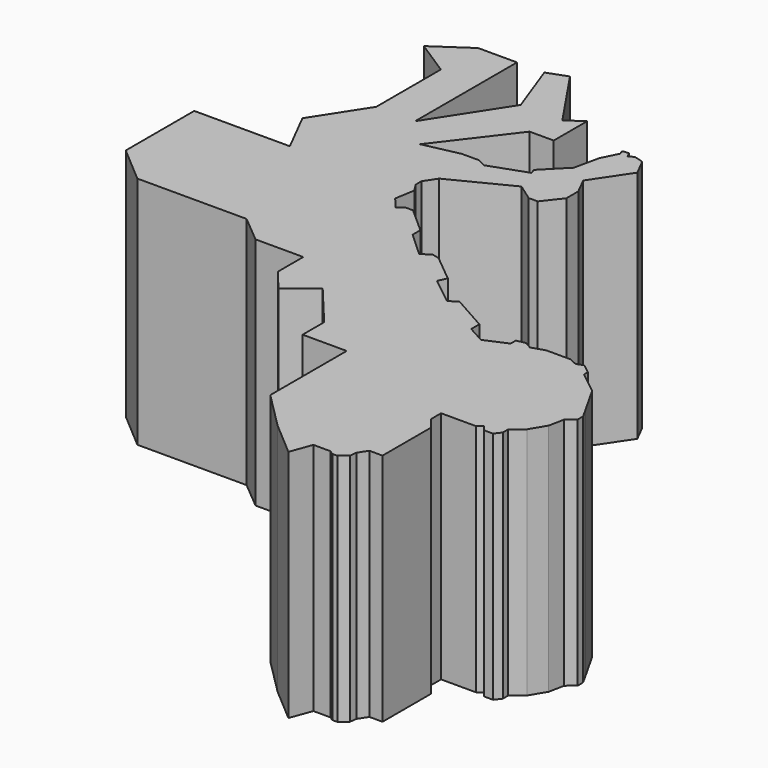
from build123d import *

# Parameters (mm, degrees)
F1_DEPTH    = 18.4
F2_T        = 1
F2_T3_DEPTH = 20.4


# Not quite as in the source:
# - a shell that OpenCascade refuses in one call is made with other operations: the cavity is built on its own and cut out


with BuildPart() as f1:
    # F0 (on Top) → F1 (new body)
    with BuildSketch(Plane.XY):
        Polygon((34.9038466811, 2.3076923098), (37.5961586833, 0), (38.2154919207, 1.6792200898), (39.5493015629, 1.6792200898), (39.8643054068, 1.4717115684), (40.2604434894, 1.4717115684), (40.8580452204, 1.969713252), (40.9277250636, 2.5216304831), (41.3846634328, 3.2152759377), (42.4140951151, 3.2152759377), (42.4140951151, 3.9669456892), (42.4140951151, 5.5783051066), (42.4140951151, 7.9888809662), (41.7042225599, 8.8407276198), (41.7042225599, 9.8502271683), (44.4576912096, 9.8502271683), (44.8243346239, 10.1557634948), (45.1803691685, 9.7285222481), (45.8762775312, 9.7285222481), (46.256152948, 10.2124772966), (46.256152948, 10.7373551534), (47.1577197313, 11.48866117), (47.8789657354, 12.6923089847), (48.1241039427, 13.9088267574), (48.7609393895, 14.4395232201), (48.7609393895, 14.9668920785), (48.3345761895, 15.7310124487), (47.0663927722, 17.9758262752), (45.3253550111, 19.3424355239), (45.3253550111, 19.7353474796), (44.5925742388, 20.310536027), (44.0478101373, 20.1109051704), (43.4293858707, 20.3982274979), (41.5340252221, 20.3982274979), (40.4943935573, 20.0712326914), (39.9509593844, 20.3926954418), (39.258543402, 20.2461257577), (39.258543402, 19.7353474796), (37.5306159258, 18.9858879894), (36.1601188779, 19.7353474796), (36.1601188779, 20.5363873392), (33.3506949246, 22.1185106784), (32.6812267303, 21.7167064548), (30.5281542242, 23.4213601798), (30.8408737183, 24.0895077586), (28.7077520043, 25.8446503431), (28.1511750072, 25.9745512158), (27.4442564696, 25.5241394043), (25.5313739181, 27.267659083), (25.5313739181, 28.0364025384), (23.5221236944, 29.8172839707), (22.9337685687, 29.8172839707), (22.4811825901, 29.4311344624), (21.6883961111, 30.3603187203), (21.9499040395, 31.9214127958), (21.5246956795, 32.5762294233), (21.5246956795, 33.1562906504), (22.1474349188, 34.1016265465), (26.7516728491, 36.4373363554), (28.0509851873, 35.5146564543), (28.7558529526, 35.5146564543), (29.8695010146, 36.9334258139), (29.8695010146, 38.1099569989), (29.2044375092, 39.4209548831), (31.1400774979, 42.3122339083), (30.4684508592, 43.6361692846), (29.7395295394, 43.846223038), (29.3254637787, 43.6361692846), (29.1439853609, 43.9939062825), (28.7558529526, 43.9939062825), (28.6115187719, 43.9206861825), (28.7558529526, 43.6361692846), (28.1240884215, 42.362369597), (27.6678408464, 40.2808707131), (27.4981055409, 40.1947647333), (25.9593750461, 38.6289927336), (26.0996799916, 38.2336303592), (23.197773844, 37.2038111091), (22.5049275905, 37.5358015299), (21.194729954, 37.5358015299), (18.3843486011, 36.9334258139), (22.5816704333, 42.4372814596), (24.4770020993, 42.4372814596), (24.4770020993, 45.7188370083), (23.2146158814, 44.8650717735), (19.9435582577, 49.7016918345), (18.3843486011, 49.1319186985), (19.9435582577, 44.8650717735), (16.2385422736, 39.1325615346), (16.2385422736, 44.8650717735), (16.2385422736, 49.1319186985), (13.1833981723, 49.1319186985), (10.4276611454, 47.2565910677), (13.1833981723, 45.475512743), (13.1833981723, 39.1325615346), (10.5969374999, 35.130713135), (12.3173817992, 31.7393094301), (8.6204865947, 31.7393094301), (4.8114596866, 31.7393094301), (4.8114596866, 28.6961421371), (4.8114596866, 25.0201616436), (7.6984064654, 22.5476305932), (11.4156892523, 22.5476305932), (16.276538372, 22.5476305932), (18.3994080871, 20.769232884), (20.5554086715, 20.769232884), (22.1474349188, 20.769232884), (22.1474349188, 18.2692315429), (23.5923715867, 16.5353083812), (25.6730783731, 18.2692315429), (28.5576954484, 14.8076927289), (28.5576954484, 12.6923089847), (32.0192314684, 12.6923089847), (32.0192314684, 5.192308221), align=None)
    extrude(amount=F1_DEPTH)

    # F2: shell of thickness 1, made by hand


with BuildPart() as f2_core1:
    # F2_t2: copy of F1
    add(f1.part)

    # the walls: a layer under each face that stays
    f2_faces = [f2_core1.faces().sort_by_distance(p)[0] for p in [
        (13.1833981723, 42.3040371388, 9.2),
        (26.786199538, 24.8508459173, 18.4),
        (11.8055296588, 48.1942548831, 9.2),
        (14.7109702229, 49.1319186985, 9.2),
        (16.2385422736, 44.1322401166, 9.2),
        (18.0910502657, 41.9988166541, 9.2),
        (19.1639534294, 46.998495236, 9.2),
        (19.1639534294, 49.4168052665, 9.2),
        (21.5790870696, 47.283381804, 9.2),
        (23.8458089904, 45.2919543909, 9.2),
        (24.4770020993, 44.0780592339, 9.2),
        (23.5293362663, 42.4372814596, 9.2),
        (20.4830095172, 39.6853536367, 9.2),
        (19.7895392776, 37.2346136719, 9.2),
        (21.8498287722, 37.5358015299, 9.2),
        (22.8513507172, 37.3698063195, 9.2),
        (24.6487269178, 37.7187207341, 9.2),
        (26.0295275188, 38.4313115464, 9.2),
        (26.7287402935, 39.4118787334, 9.2),
        (27.5829731936, 40.2378177232, 9.2),
        (27.8959646339, 41.321620155, 9.2),
        (28.439970687, 42.9992694408, 9.2),
        (28.6836858623, 43.7784277335, 9.2),
        (28.6836858623, 43.9572962325, 9.2),
        (28.9499191567, 43.9939062825, 9.2),
        (29.2347245698, 43.8150377835, 9.2),
        (29.5324966591, 43.7411961613, 9.2),
        (30.1039901993, 43.7411961613, 9.2),
        (30.8042641785, 42.9742015964, 9.2),
        (30.1722575035, 40.8665943957, 9.2),
        (29.5369692619, 38.765455941, 9.2),
        (29.8695010146, 37.5216914064, 9.2),
        (29.3126769836, 36.2240411341, 9.2),
        (28.4034190699, 35.5146564543, 9.2),
        (27.4013290182, 35.9759964049, 9.2),
        (24.4495538839, 35.269481451, 9.2),
        (21.8360652992, 33.6289585984, 9.2),
        (21.5246956795, 32.8662600368, 9.2),
        (21.7372998595, 32.2488211095, 9.2),
        (21.8191500753, 31.1408657581, 9.2),
        (22.0847893506, 29.8957265913, 9.2),
        (22.7074755794, 29.6242092165, 9.2),
        (23.2279461315, 29.8172839707, 9.2),
        (24.5267488062, 28.9268432546, 9.2),
        (25.5313739181, 27.6520308107, 9.2),
        (26.4878151938, 26.3958992437, 9.2),
        (27.7977157384, 25.74934531, 9.2),
        (28.4294635057, 25.9096007794, 9.2),
        (29.7743128613, 24.9670790508, 9.2),
        (30.6845139712, 23.7554339692, 9.2),
        (31.6046904773, 22.5690333173, 9.2),
        (33.0159608275, 21.9176085666, 9.2),
        (34.7554069012, 21.3274490088, 9.2),
        (36.1601188779, 20.1358674094, 9.2),
        (36.8453674018, 19.3606177345, 9.2),
        (38.3945796639, 19.3606177345, 9.2),
        (39.258543402, 19.9907366186, 9.2),
        (39.6047513932, 20.3194105998, 9.2),
        (40.2226764709, 20.2319640666, 9.2),
        (41.0142093897, 20.2347300947, 9.2),
        (42.4817055464, 20.3982274979, 9.2),
        (43.738598004, 20.2545663342, 9.2),
        (44.320192188, 20.2107205987, 9.2),
        (44.958964625, 20.0229417533, 9.2),
        (45.3253550111, 19.5388915017, 9.2),
        (46.1958738917, 18.6591308995, 9.2),
        (47.7004844809, 16.8534193619, 9.2),
        (48.5477577895, 15.3489522636, 9.2),
        (48.7609393895, 14.7032076493, 9.2),
        (48.4425216661, 14.1741749888, 9.2),
        (48.0015348391, 13.3005678711, 9.2),
        (47.5183427334, 12.0904850774, 9.2),
        (46.7069363397, 11.1130081617, 9.2),
        (46.256152948, 10.474916225, 9.2),
        (46.0662152396, 9.9704997724, 9.2),
        (45.5283233499, 9.7285222481, 9.2),
        (45.0023518962, 9.9421428715, 9.2),
        (44.6410129167, 10.0029953316, 9.2),
        (43.0809568847, 9.8502271683, 9.2),
        (41.7042225599, 9.3454773941, 9.2),
        (42.0591588375, 8.414804293, 9.2),
        (42.4140951151, 5.6020784519, 9.2),
        (41.899379274, 3.2152759377, 9.2),
        (41.1561942482, 2.8684532104, 9.2),
        (40.892885142, 2.2456718676, 9.2),
        (40.5592443549, 1.7207124102, 9.2),
        (40.0623744481, 1.4717115684, 9.2),
        (39.7068034849, 1.5754658291, 9.2),
        (38.8823967418, 1.6792200898, 9.2),
        (37.905825302, 0.8396100449, 9.2),
        (36.2500026822, 1.1538461549, 9.2),
        (33.4615390748, 3.7500002654, 9.2),
        (32.0192314684, 8.9423086029, 9.2),
        (30.2884634584, 12.6923089847, 9.2),
        (28.5576954484, 13.7500008568, 9.2),
        (27.1153869107, 16.5384621359, 9.2),
        (24.6327249799, 17.4022699621, 9.2),
        (22.8699032528, 17.4022699621, 9.2),
        (22.1474349188, 19.5192322135, 9.2),
        (20.273421503, 20.769232884, 9.2),
        (17.3379732296, 21.6584317386, 9.2),
        (11.9874724187, 22.5476305932, 9.2),
        (6.254933076, 23.7838961184, 9.2),
        (4.8114596866, 28.3797355369, 9.2),
        (8.5644207429, 31.7393094301, 9.2),
        (11.4571596496, 33.4350112826, 9.2),
        (11.8901678361, 37.1316373348, 9.2),
        (11.8055296588, 46.3660519053, 9.2),
    ]]
    thicken(f2_faces, amount=-F2_T, mode=Mode.SUBTRACT)

    # F2_s4 → F2_t3 (cut)
    with BuildSketch(Plane.XY.offset(-1)):
        Polygon((13.1679700547, 45.4671141991), (14.1833981723, 45.475512743), (14.1833981723, 46.0198788256), (13.7262099274, 46.3153671343), align=None)
        Polygon((13.1649996283, 39.1379896522), (14.1833981723, 39.1325615346), (14.1833981723, 38.8375317988), (14.0232525635, 38.5897497795), align=None)
        Polygon((16.2401437297, 39.1379896522), (15.2385422736, 39.1325615346), (15.2385422736, 35.7430726852), (17.0783966649, 38.5897497795), align=None)
        Polygon((19.9257671848, 44.8670676325), (20.783412649, 44.3222600184), (21.0537457725, 44.7405274174), (20.8828111582, 45.2082976305), align=None)
        Polygon((23.2172971457, 44.8789574072), (22.3862709855, 44.3048533043), (22.9464894547, 43.4765084083), (23.7748343507, 44.0367268776), align=None)
        Polygon((22.5896220279, 42.4212174557), (22.5816704333, 43.4372814596), (22.0866758653, 43.4372814596), (21.786510969, 43.0436818441), align=None)
        Polygon((18.3902044021, 36.9371397265), (17.5891891368, 37.5398261984), (15.9486712075, 35.3886511806), (18.5939279659, 35.9556341746), align=None)
        Polygon((23.1987506451, 37.2222534255), (22.7656519794, 36.3019958873), (23.1404957465, 36.1223823882), (23.5322155954, 36.2613946858), align=None)
        Polygon((26.0869114099, 38.2397101059), (26.434121743, 37.2912139359), (27.3765381663, 37.6256556872), (27.0420964149, 38.5680721106), align=None)
        Polygon((27.6535486373, 40.2919298957), (28.1202519233, 39.3890611945), (28.5431256697, 39.6035832006), (28.6446506768, 40.0667619668), align=None)
        Polygon((28.7379761854, 43.636088393), (29.6517201492, 43.1918473673), (29.8746005614, 43.641231569), (29.6476624712, 44.0885803615), align=None)
        Polygon((29.3298577631, 43.6496114905), (28.4336542601, 43.1837582077), (28.886065337, 42.2919486891), (29.7778748556, 42.744359766), align=None)
        Polygon((29.2216653197, 39.4199158444), (28.3734659785, 39.9772698255), (28.0477314009, 39.4907178027), (28.3126279906, 38.9685438062), align=None)
        Polygon((26.7504070392, 36.4202649285), (27.3306649145, 37.2526695316), (26.838065671, 37.6024787406), (26.2992617722, 37.3291458741), align=None)
        Polygon((22.1603099227, 34.0872073074), (21.6950238419, 34.9934360651), (21.4583427741, 34.8733687923), (21.3123456088, 34.6517409384), align=None)
        Polygon((21.5430465726, 33.1507895064), (20.6896063695, 33.7064050423), (20.5246956795, 33.4560659196), (20.5246956795, 33.1562906504), align=None)
        Polygon((21.5430825872, 32.5816755026), (20.5246956795, 32.5762294233), (20.5246956795, 32.2800361011), (20.6860049108, 32.031621496), align=None)
        Polygon((21.7058660301, 30.3651572191), (20.7021383294, 30.5255324851), (20.6251317696, 30.0658352013), (20.9276619991, 29.7112550788), align=None)
        Polygon((22.4822992948, 29.4452324399), (21.7204484781, 28.7820708208), (22.3695121196, 28.0213367088), (23.1302462317, 28.6704003503), align=None)
        Polygon((25.5481102347, 27.2750497553), (24.5313739181, 27.267659083), (24.5313739181, 26.8260641688), (24.8577422495, 26.5285918498), align=None)
        Polygon((27.4456193232, 25.5399636935), (26.7706248011, 24.7850721711), (27.3362073239, 24.2695652166), (27.9816027793, 24.6807777123), align=None)
        Polygon((30.5434186232, 23.4249613309), (29.6224481569, 23.8452664426), (29.2869956516, 23.1285481585), (29.9074203913, 22.6373388097), align=None)
        Polygon((32.6822879499, 21.7331209009), (32.0604928975, 20.9326850846), (32.6027806407, 20.5033391993), (33.1958386031, 20.8592832101), align=None)
        Polygon((36.1749168481, 19.7441212747), (35.1601188779, 19.7353474796), (35.1601188779, 19.1424421675), (35.6803218539, 18.8579679632), align=None)
        Polygon((37.5314347335, 19.003836002), (37.0508189018, 18.108508473), (37.4798845986, 17.8738729013), (37.9285321814, 18.068466247), align=None)
        Polygon((39.2445642394, 19.744521697), (39.6564596576, 18.8179257372), (40.258543402, 19.0790694381), (40.258543402, 19.7353474796), align=None)
        Polygon((40.496484489, 20.0893788513), (39.9852621723, 19.2105438784), (40.3690586499, 18.9835131221), (40.7944317772, 19.1173055104), align=None)
        Polygon((44.0485828398, 20.1293635667), (43.6264614535, 19.2040064514), (44.0025314328, 19.0292828714), (44.3918885697, 19.1719642605), align=None)
        Polygon((45.3415294575, 19.3503016673), (44.3253550111, 19.3424355239), (44.3253550111, 18.8561039856), (44.7079103727, 18.5558211848), align=None)
        Polygon((48.1403087419, 13.8991691715), (47.4839193601, 14.6770478846), (47.2133752837, 14.4515943784), (47.1438086054, 14.1063642263), align=None)
        Polygon((46.2725547938, 10.7296729421), (45.6159683654, 11.5055762805), (45.256152948, 11.2057299542), (45.256152948, 10.7373551534), align=None)
        Polygon((44.8230542584, 10.1416794377), (45.592555751, 10.7959480775), (44.9523711683, 11.5641692046), (44.1841500412, 10.923984622), align=None)
        Polygon((41.7142225599, 9.8402271683), (41.7042225599, 10.8502271683), (40.7042225599, 10.8502271683), (40.7042225599, 9.8502271683), align=None)
        Polygon((41.7219047712, 8.8471294657), (40.7042225599, 8.8407276198), (40.7042225599, 8.4786775499), (40.9360014328, 8.2005430372), align=None)
        Polygon((41.3930143259, 3.1997747938), (41.3846634328, 4.2152759377), (40.8459358948, 4.2152759377), (40.5495741228, 3.7653903296), align=None)
        Polygon((40.945997201, 2.5148767768), (40.0926357536, 3.071744875), (39.9647248354, 2.8775724593), (39.9356006382, 2.6468867182), align=None)
        Polygon((39.543800419, 1.6608691967), (40.0994159549, 2.5143093999), (39.8490768321, 2.6792200898), (39.5493015629, 2.6792200898), align=None)
        Polygon((38.2248741311, 1.6657597246), (38.2154919207, 2.6792200898), (37.5184669666, 2.6792200898), (37.2772708771, 2.0252566099), align=None)
        Polygon((32.0092314684, 12.6823089847), (33.0192314684, 12.6923089847), (33.0192314684, 13.6923089847), (32.0192314684, 13.6923089847), align=None)
        Polygon((28.5400132371, 14.8012908831), (29.5576954484, 14.8076927289), (29.5576954484, 15.1697427988), (29.3259165755, 15.4478773116), align=None)
        Polygon((25.6717980076, 18.2551474858), (26.4412995002, 18.9094161256), (25.8011149176, 19.6776372527), (25.0328937904, 19.0374526701), align=None)
        Polygon((22.1374349188, 20.759232884), (23.1474349188, 20.769232884), (23.1474349188, 21.769232884), (22.1474349188, 21.769232884), align=None)
        Polygon((16.2701166463, 22.5299649922), (16.9187109501, 23.3141906887), (16.6400542126, 23.5476305932), (16.276538372, 23.5476305932), align=None)
        Polygon((12.308463704, 31.7447853194), (12.3173817992, 30.7393094301), (13.9459931188, 30.7393094301), (13.2091913178, 32.191720507), align=None)
    extrude(amount=F2_T3_DEPTH, mode=Mode.SUBTRACT)


with BuildPart() as f1_1:
    add(f1.part)

    # what is left inside the walls is the cavity
    f2_cavity = [f2_core1.part.solids().sort_by_distance(p)[0] for p in [
        (16.279679, 32.652899, 17.39),
        (27.61088, 38.86856, 11.6),
        (29.357123, 41.464541, 11.6),
    ]]
    add(f2_cavity, mode=Mode.SUBTRACT)


solid = f1_1.part
